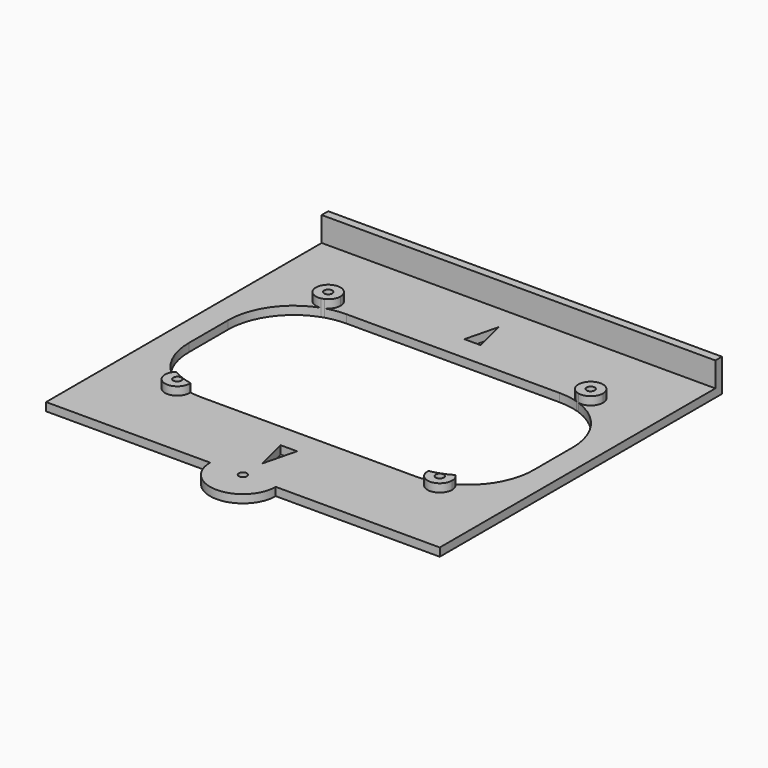
from build123d import *

# Parameters (mm, degrees)
F0_R     = 1.5875
F0_W     = 152.4
F0_H     = 3.175
F1_DEPTH = 3.175
F2_DEPTH = 6.35
F3_DEPTH = 12.7


# Not quite as in the source:
# - a feature names something its author has since deleted; it is built from what else it names


with BuildPart() as f1:
    # F0 (on Top) → F1 (new body)
    with BuildSketch(Plane.XY):
        with BuildLine():
            Line((76.2, -63.5), (76.2, 60.325))
            Line((76.2, 60.325), (-76.2, 60.325))
            Line((-76.2, 60.325), (-76.2, -63.5))
            Line((-76.2, -63.5), (-76.2, -73.025))
            Line((-76.2, -73.025), (-12.7, -73.025))
            ThreePointArc((-12.7, -73.025), (0, -85.725), (12.7, -73.025))
            Line((12.7, -73.025), (76.2, -73.025))
            Line((76.2, -73.025), (76.2, -63.5))
        make_face()
        with Locations((0, -73.025)):
            Circle(F0_R, mode=Mode.SUBTRACT)
        Polygon((3.175, -50.8), (0, -63.5), (-3.175, -50.8), align=None, mode=Mode.SUBTRACT)
        with BuildLine():
            ThreePointArc((-49.8535963292, 27.0824817792), (-54.4870485305, 34.7644782938), (-46.0375, 31.75))
            ThreePointArc((-46.0375, 31.75), (-46.7742676703, 29.2054203766), (-48.7566120041, 27.4481432208))
            ThreePointArc((-48.7566120041, 27.4481432208), (-45.0579989552, 28.2917059724), (-41.275, 28.575))
            Line((-41.275, 28.575), (41.275, 28.575))
            ThreePointArc((41.275, 28.575), (45.0579989552, 28.2917059724), (48.7566120041, 27.4481432208))
            ThreePointArc((48.7566120041, 27.4481432208), (48.2554203766, 35.7757323297), (55.5625, 31.75))
            ThreePointArc((55.5625, 31.75), (53.8144782938, 28.0629514695), (49.8535963292, 27.0824817792))
            ThreePointArc((49.8535963292, 27.0824817792), (62.0482562055, 17.7911495141), (66.675, 3.175))
            Line((66.675, 3.175), (66.675, -15.875))
            ThreePointArc((66.675, -15.875), (63.3002757063, -28.525977435), (54.0728559007, -37.8152571622))
            ThreePointArc((54.0728559007, -37.8152571622), (55.1742646512, -39.3915948361), (55.5625, -41.275))
            ThreePointArc((55.5625, -41.275), (50.5724196506, -46.0320593264), (46.0592502637, -40.8203592761))
            ThreePointArc((46.0592502637, -40.8203592761), (43.6779018277, -41.1610843708), (41.275, -41.275))
            Line((41.275, -41.275), (-41.275, -41.275))
            ThreePointArc((-41.275, -41.275), (-43.6779018277, -41.1610843708), (-46.0592502637, -40.8203592761))
            ThreePointArc((-46.0592502637, -40.8203592761), (-46.0429406736, -41.0474196506), (-46.0375, -41.275))
            ThreePointArc((-46.0375, -41.275), (-52.6834051639, -45.6492646512), (-54.0728559007, -37.8152571622))
            ThreePointArc((-54.0728559007, -37.8152571622), (-63.3002757063, -28.525977435), (-66.675, -15.875))
            Line((-66.675, -15.875), (-66.675, 3.175))
            ThreePointArc((-66.675, 3.175), (-62.0482562055, 17.7911495141), (-49.8535963292, 27.0824817792))
        make_face(mode=Mode.SUBTRACT)
        Polygon((-3.175, 38.1), (0, 50.8), (3.175, 38.1), align=None, mode=Mode.SUBTRACT)
        with Locations((0, 61.9125)):
            Rectangle(F0_W, F0_H)
        with BuildLine():
            ThreePointArc((-48.7566120041, 27.4481432208), (-46.7742676703, 29.2054203766), (-46.0375, 31.75))
            ThreePointArc((-46.0375, 31.75), (-54.4870485305, 34.7644782938), (-49.8535963292, 27.0824817792))
            ThreePointArc((-49.8535963292, 27.0824817792), (-49.3071852568, 27.2715557705), (-48.7566120041, 27.4481432208))
        make_face()
        with Locations((-50.8, 31.75)):
            Circle(F0_R, mode=Mode.SUBTRACT)
        with BuildLine():
            ThreePointArc((55.5625, 31.75), (48.2554203766, 35.7757323297), (48.7566120041, 27.4481432208))
            ThreePointArc((48.7566120041, 27.4481432208), (49.3071852568, 27.2715557705), (49.8535963292, 27.0824817792))
            ThreePointArc((49.8535963292, 27.0824817792), (53.8144782938, 28.0629514695), (55.5625, 31.75))
        make_face()
        with Locations((50.8, 31.75)):
            Circle(F0_R, mode=Mode.SUBTRACT)
        with BuildLine():
            ThreePointArc((54.0728559007, -37.8152571622), (50.1935354163, -39.6577611103), (46.0592502637, -40.8203592761))
            ThreePointArc((46.0592502637, -40.8203592761), (50.5724196506, -46.0320593264), (55.5625, -41.275))
            ThreePointArc((55.5625, -41.275), (55.1742646512, -39.3915948361), (54.0728559007, -37.8152571622))
        make_face()
        with Locations((50.8, -41.275)):
            Circle(F0_R, mode=Mode.SUBTRACT)
        with BuildLine():
            ThreePointArc((-46.0592502637, -40.8203592761), (-50.1935354163, -39.6577611103), (-54.0728559007, -37.8152571622))
            ThreePointArc((-54.0728559007, -37.8152571622), (-52.6834051639, -45.6492646512), (-46.0375, -41.275))
            ThreePointArc((-46.0375, -41.275), (-46.0429406736, -41.0474196506), (-46.0592502637, -40.8203592761))
        make_face()
        with Locations((-50.8, -41.275)):
            Circle(F0_R, mode=Mode.SUBTRACT)
    extrude(amount=F1_DEPTH)

    # F0 (on Top) → F2 (join)
    with BuildSketch(Plane.XY):
        with BuildLine():
            ThreePointArc((-46.0592502637, -40.8203592761), (-50.1935354163, -39.6577611103), (-54.0728559007, -37.8152571622))
            ThreePointArc((-54.0728559007, -37.8152571622), (-52.6834051639, -45.6492646512), (-46.0375, -41.275))
            ThreePointArc((-46.0375, -41.275), (-46.0429406736, -41.0474196506), (-46.0592502637, -40.8203592761))
        make_face()
        with Locations((-50.8, -41.275)):
            Circle(F0_R, mode=Mode.SUBTRACT)
        with BuildLine():
            ThreePointArc((-48.7566120041, 27.4481432208), (-46.7742676703, 29.2054203766), (-46.0375, 31.75))
            ThreePointArc((-46.0375, 31.75), (-54.4870485305, 34.7644782938), (-49.8535963292, 27.0824817792))
            ThreePointArc((-49.8535963292, 27.0824817792), (-49.3071852568, 27.2715557705), (-48.7566120041, 27.4481432208))
        make_face()
        with Locations((-50.8, 31.75)):
            Circle(F0_R, mode=Mode.SUBTRACT)
        with BuildLine():
            ThreePointArc((54.0728559007, -37.8152571622), (50.1935354163, -39.6577611103), (46.0592502637, -40.8203592761))
            ThreePointArc((46.0592502637, -40.8203592761), (50.5724196506, -46.0320593264), (55.5625, -41.275))
            ThreePointArc((55.5625, -41.275), (55.1742646512, -39.3915948361), (54.0728559007, -37.8152571622))
        make_face()
        with Locations((50.8, -41.275)):
            Circle(F0_R, mode=Mode.SUBTRACT)
        with BuildLine():
            ThreePointArc((55.5625, 31.75), (48.2554203766, 35.7757323297), (48.7566120041, 27.4481432208))
            ThreePointArc((48.7566120041, 27.4481432208), (49.3071852568, 27.2715557705), (49.8535963292, 27.0824817792))
            ThreePointArc((49.8535963292, 27.0824817792), (53.8144782938, 28.0629514695), (55.5625, 31.75))
        make_face()
        with Locations((50.8, 31.75)):
            Circle(F0_R, mode=Mode.SUBTRACT)
    extrude(amount=F2_DEPTH)

    # F0 (on Top) → F3 (join)
    with BuildSketch(Plane.XY):
        with Locations((0, 61.9125)):
            Rectangle(F0_W, F0_H)
    extrude(amount=F3_DEPTH)


solid = f1.part
